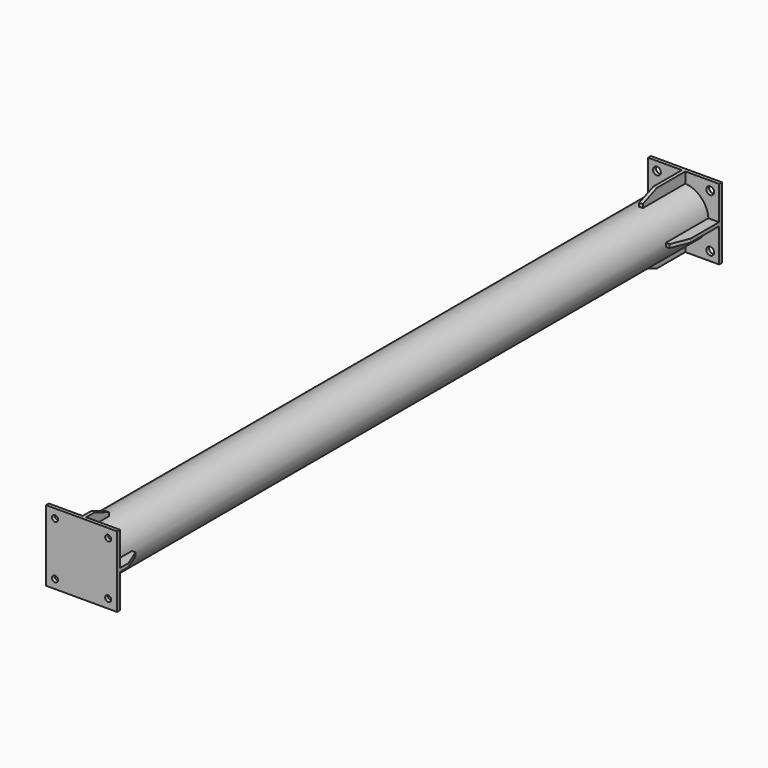
from build123d import *

# Parameters (mm, degrees)
F0_R          = 70
F0_R_2        = 65
F1_DEPTH      = 2110
F2_W          = 200
F2_H          = 200
F2_R          = 11
F3_DEPTH      = 10
F4_W          = 30.1787997812
F4_H          = 10
F4_W_2        = 10
F4_H_2        = 30.1787997812
F5_DEPTH      = 150
F6_T1_DEPTH   = 269.311363913
F6_T3_DEPTH   = 269.311363913
F6_T8_DEPTH   = 269.311363913
F6_S9_R       = 70
F6_T10_DEPTH  = 139
F8_W          = 200
F8_H          = 200
F8_R          = 8.5
F9_DEPTH      = 10
F10_W         = 10
F10_H         = 30.1787997812
F10_W_2       = 30.1787997812
F10_H_2       = 10
F11_DEPTH     = 80
F12_T1_DEPTH  = 269.311363913
F12_T3_DEPTH  = 269.311363913
F12_T8_DEPTH  = 269.311363913
F12_S9_R      = 70
F12_T10_DEPTH = 139
F12_T14_DEPTH = 269.311363913
F12_S15_R     = 70
F12_T16_DEPTH = 139


# Not quite as in the source:
# - a fillet or chamfer that OpenCascade refuses, or shapes differently, is made with other operations: its cross-section is extruded or revolved along the edge and cut away or added


with BuildPart() as f1:
    # F0 (on Front) → F1 (new body)
    with BuildSketch(Plane.XZ):
        Circle(F0_R)
        Circle(F0_R_2, mode=Mode.SUBTRACT)
    extrude(amount=F1_DEPTH)

    # F2 (on Front) → F3 (join)
    with BuildSketch(Plane.XZ):
        Rectangle(F2_W, F2_H)
        with Locations((-75, -75)):
            Circle(F2_R, mode=Mode.SUBTRACT)
        with Locations((75, -75)):
            Circle(F2_R, mode=Mode.SUBTRACT)
        with Locations((-75, 75)):
            Circle(F2_R, mode=Mode.SUBTRACT)
        with Locations((75, 75)):
            Circle(F2_R, mode=Mode.SUBTRACT)
    extrude(amount=-F3_DEPTH)

    # F4 (on Front) → F5 (join)
    with BuildSketch(Plane.XZ):
        with Locations((-84.9106001094, 0)):
            Rectangle(F4_W, F4_H)
        with Locations((0, 84.9106001094)):
            Rectangle(F4_W_2, F4_H_2)
        with Locations((84.9106001094, 0)):
            Rectangle(F4_W, F4_H)
        with Locations((0, -84.9106001094)):
            Rectangle(F4_W_2, F4_H_2)
    extrude(amount=F5_DEPTH)

    # F6: chamfer of 50 x 20 on 4 edges, made by hand

    # F6_s2 → F6_t1 (cut)
    with BuildSketch(Plane.YZ.offset(-134.6556819565)):
        Polygon((-100, 100), (-150, 80), (-150, 100), align=None)
        Polygon((-100, -100), (-150, -80), (-150, -100), align=None)
    extrude(amount=F6_T1_DEPTH, mode=Mode.SUBTRACT)

    # F6_s4 → F6_t3 (cut)
    with BuildSketch(Plane.XY.offset(-134.6556819565)):
        Polygon((100, -100), (80, -150), (100, -150), align=None)
    extrude(amount=F6_T3_DEPTH, mode=Mode.SUBTRACT)


with BuildPart() as f6_tool6:
    # F6_s7 → F6_t8 (new body)
    with BuildSketch(Plane.XY.offset(134.6556819565)):
        Polygon((-100, -130), (-50, -150), (-100, -150), align=None)
    extrude(amount=-F6_T8_DEPTH)

    # F6_s9 → F6_t10 (cut, symmetric)
    with BuildSketch(Plane.XZ.offset(140)):
        Circle(F6_S9_R)
    extrude(amount=F6_T10_DEPTH, both=True, mode=Mode.SUBTRACT)


with BuildPart() as f1_1:
    add(f1.part)

    # F6_t5: cut F6_tool6
    add(f6_tool6.part, mode=Mode.SUBTRACT)

    # F8 (on offset) → F9 (join)
    with BuildSketch(Plane.XZ.offset(2110)):
        Rectangle(F8_W, F8_H)
        with Locations((-75, -75)):
            Circle(F8_R, mode=Mode.SUBTRACT)
        with Locations((75, -75)):
            Circle(F8_R, mode=Mode.SUBTRACT)
        with Locations((-75, 75)):
            Circle(F8_R, mode=Mode.SUBTRACT)
        with Locations((75, 75)):
            Circle(F8_R, mode=Mode.SUBTRACT)
    extrude(amount=F9_DEPTH)

    # F10 (on face) → F11 (join)
    with BuildSketch(Plane(origin=(0, -2110, 0), x_dir=(-1, 0, 0), z_dir=(0, 1, 0))):
        with Locations((0, 84.9106001094)):
            Rectangle(F10_W, F10_H)
        with Locations((84.9106001094, 0)):
            Rectangle(F10_W_2, F10_H_2)
        with Locations((0, -84.9106001094)):
            Rectangle(F10_W, F10_H)
        with Locations((-84.9106001094, 0)):
            Rectangle(F10_W_2, F10_H_2)
    extrude(amount=F11_DEPTH)

    # F12: chamfer of 20 x 50 on 4 edges, made by hand

    # F12_s2 → F12_t1 (cut)
    with BuildSketch(Plane.YZ.offset(-134.6556819565)):
        Polygon((-2080, 100), (-2030, 80), (-2030, 100), align=None)
    extrude(amount=F12_T1_DEPTH, mode=Mode.SUBTRACT)

    # F12_s4 → F12_t3 (cut)
    with BuildSketch(Plane.XY.offset(-134.6556819565)):
        Polygon((100, -2080), (80, -2030), (100, -2030), align=None)
    extrude(amount=F12_T3_DEPTH, mode=Mode.SUBTRACT)


with BuildPart() as f12_tool6:
    # F12_s7 → F12_t8 (new body)
    with BuildSketch(Plane.XY.offset(-134.6556819565)):
        Polygon((-100, -2050), (-50, -2030), (-100, -2030), align=None)
    extrude(amount=F12_T8_DEPTH)

    # F12_s9 → F12_t10 (cut, symmetric)
    with BuildSketch(Plane.XZ.offset(2040)):
        Circle(F12_S9_R)
    extrude(amount=F12_T10_DEPTH, both=True, mode=Mode.SUBTRACT)


with BuildPart() as f1_2:
    add(f1_1.part)

    # F12_t5: cut F12_tool6
    add(f12_tool6.part, mode=Mode.SUBTRACT)


with BuildPart() as f12_tool12:
    # F12_s13 → F12_t14 (new body)
    with BuildSketch(Plane.YZ.offset(134.6556819565)):
        Polygon((-2050, -100), (-2030, -50), (-2030, -100), align=None)
    extrude(amount=-F12_T14_DEPTH)

    # F12_s15 → F12_t16 (cut, symmetric)
    with BuildSketch(Plane.XZ.offset(2040)):
        Circle(F12_S15_R)
    extrude(amount=F12_T16_DEPTH, both=True, mode=Mode.SUBTRACT)


with BuildPart() as f1_3:
    add(f1_2.part)

    # F12_t11: cut F12_tool12
    add(f12_tool12.part, mode=Mode.SUBTRACT)


solid = f1_3.part
